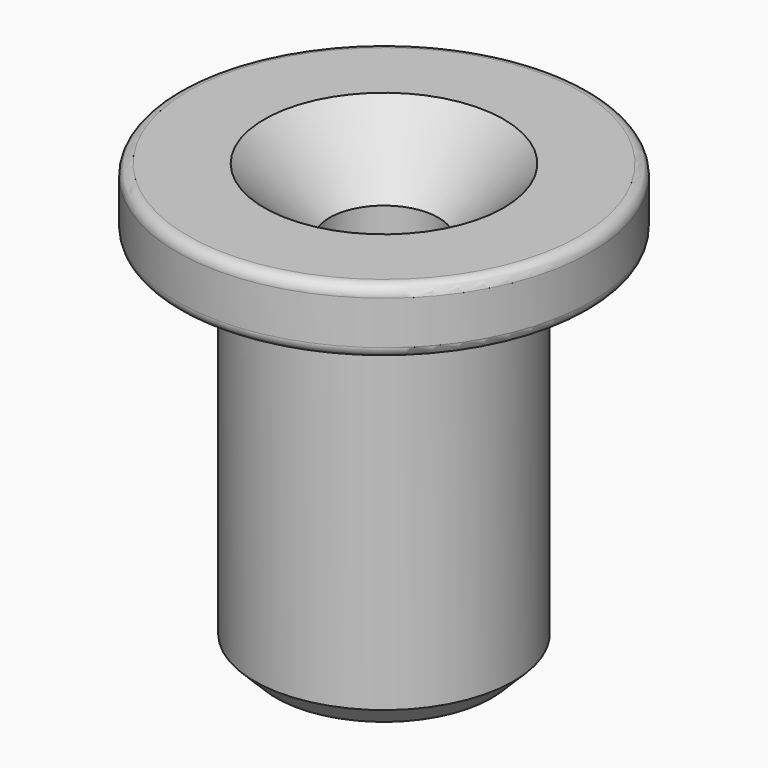
from build123d import *

# Parameters (mm, degrees)
F0_R     = 9.5
F0_R_2   = 2.5
F1_DEPTH = 3
F2_SIZE  = 2.99999
F3_R     = 5.95
F3_R_2   = 2.5
F4_DEPTH = 17
F5_SIZE  = 1
F6_R     = 0.5


# Not quite as in the source:
# - a fillet or chamfer is up to 0.001 mm smaller than in the source, because OpenCascade refuses the exact size
# - a feature names something its author has since deleted; it is built from what else it names


with BuildPart() as f1:
    # F0 (on Top) → F1 (new body)
    with BuildSketch(Plane.XY):
        with Locations((-18.3589216322, 16.7421158403)):
            Circle(F0_R)
        with Locations((-18.3589216322, 16.7421158403)):
            Circle(F0_R_2, mode=Mode.SUBTRACT)
    extrude(amount=F1_DEPTH)

    # F2 (size 3 in the source; OpenCascade refuses exactly that, so slightly less here)
    f2_edges = [f1.edges().sort_by_distance(p)[0] for p in [
        (-20.858922, 16.742116, 3),
    ]]
    chamfer(f2_edges, length=F2_SIZE)

    # F3 (on face) → F4 (join)
    with BuildSketch(Plane(origin=(0, 0, 0), x_dir=(1, 0, 0), z_dir=(0, 0, -1))):
        with Locations((-18.3589216322, -16.7421158403)):
            Circle(F3_R)
        with Locations((-18.3589216322, -16.7421158403)):
            Circle(F3_R_2, mode=Mode.SUBTRACT)
    extrude(amount=F4_DEPTH)

    # F5
    f5_edges = [f1.edges().sort_by_distance(p)[0] for p in [
        (-24.308922, 16.742116, -17),
    ]]
    chamfer(f5_edges, length=F5_SIZE)

    # F6
    f6_edges = [f1.edges().sort_by_distance(p)[0] for p in [
        (-27.858922, 16.742116, 0),
        (-27.858922, 16.742116, 3),
        (-24.308922, 16.742116, 0),
    ]]
    fillet(f6_edges, radius=F6_R)


solid = f1.part
